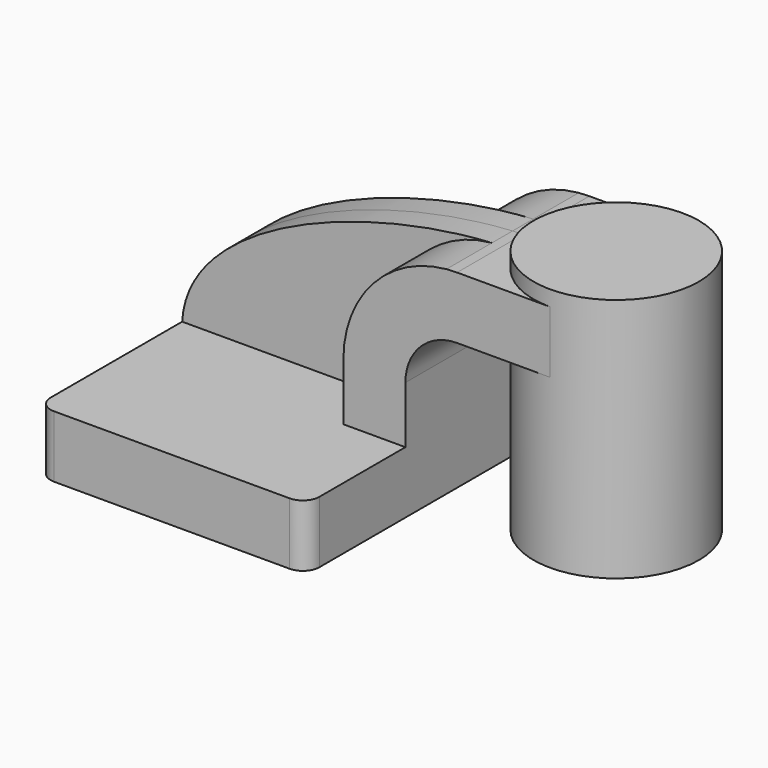
from build123d import *

# Parameters (mm, degrees)
F1_DEPTH = 63.5
F0_W     = 25.4
F0_H     = 19.05
F2_DEPTH = 25.4
F3_DEPTH = 7.9375
F5_R     = 5.08
F6_DEPTH = 46.736


with BuildPart() as f1:
    # F0 (on Front) → F1 (new body, symmetric)
    with BuildSketch(Plane.XZ):
        Polygon((22.225, 9.525), (-41.275, 9.525), (-41.275, -9.525), (41.275, -9.525), (41.275, 9.525), align=None)
    extrude(amount=F1_DEPTH, both=True)

    # F0 (on Front) → F2 (join, symmetric)
    with BuildSketch(Plane.XZ):
        with BuildLine():
            Line((22.225, 27.0002), (22.225, 9.525))
            Line((22.225, 9.525), (41.275, 9.525))
            Line((41.275, 9.525), (41.275, 27.0002))
            ThreePointArc((41.275, 27.0002), (45.9246798487, 38.2255201513), (57.15, 42.8752))
            Line((57.15, 42.8752), (60.325, 42.8752))
            Line((60.325, 42.8752), (60.325, 61.9252))
            Line((60.325, 61.9252), (57.15, 61.9252))
            add(Edge.make_bspline(
                [(53.8854342407, 61.7722898912), (54.9842067368, 61.8365871986), (56.0728453275, 61.8876096574), (57.15, 61.9252)],
                knots=[108.5245810491, 108.5245810491, 108.5245810491, 108.5245810491, 111.5045361635, 111.5045361635, 111.5045361635, 111.5045361635], degree=3))
            ThreePointArc((53.8854342407, 61.7722898912), (31.3258777096, 50.5133948686), (22.225, 27.0002))
        make_face()
        with Locations((73.025, 52.4002)):
            Rectangle(F0_W, F0_H)
    extrude(amount=F2_DEPTH, both=True)

    # F0 (on Front) → F3 (join, symmetric)
    with BuildSketch(Plane.XZ):
        with BuildLine():
            add(Edge.make_bspline(
                [(-41.275, 9.525), (-39.5856284224, 39.4828766469), (13.870125209, 59.4306981306), (53.8854342407, 61.7722898912)],
                knots=[0, 0, 0, 0, 108.5245810491, 108.5245810491, 108.5245810491, 108.5245810491], degree=3))
            Line((-41.275, 9.525), (22.225, 9.525))
            Line((22.225, 9.525), (22.225, 27.0002))
            ThreePointArc((22.225, 27.0002), (31.3258777096, 50.5133948686), (53.8854342407, 61.7722898912))
        make_face()
    extrude(amount=F3_DEPTH, both=True)

    # F0 (on Front) → F4 (revolve)
    with BuildSketch(Plane.XZ):
        Polygon((85.725, 66.675), (85.725, 61.9252), (85.725, 42.8752), (85.725, 38.1), (111.125, 38.1), (111.125, 66.675), align=None)
    revolve(axis=Axis((85.725, 0, 52.3875), (0, 0, 1)))

    # F5
    f5_edges = [f1.edges().sort_by_distance(p)[0] for p in [
        (41.275, -63.5, 0),
        (-41.275, -63.5, 0),
        (41.275, 63.5, 0),
        (-41.275, 63.5, 0),
    ]]
    fillet(f5_edges, radius=F5_R)

    # F6 (add): a face of the model
    f6_faces = [f1.faces().sort_by_distance(p)[0] for p in [
        (85.725, 0, 38.1),
    ]]
    extrude(f6_faces, amount=F6_DEPTH)


solid = f1.part
